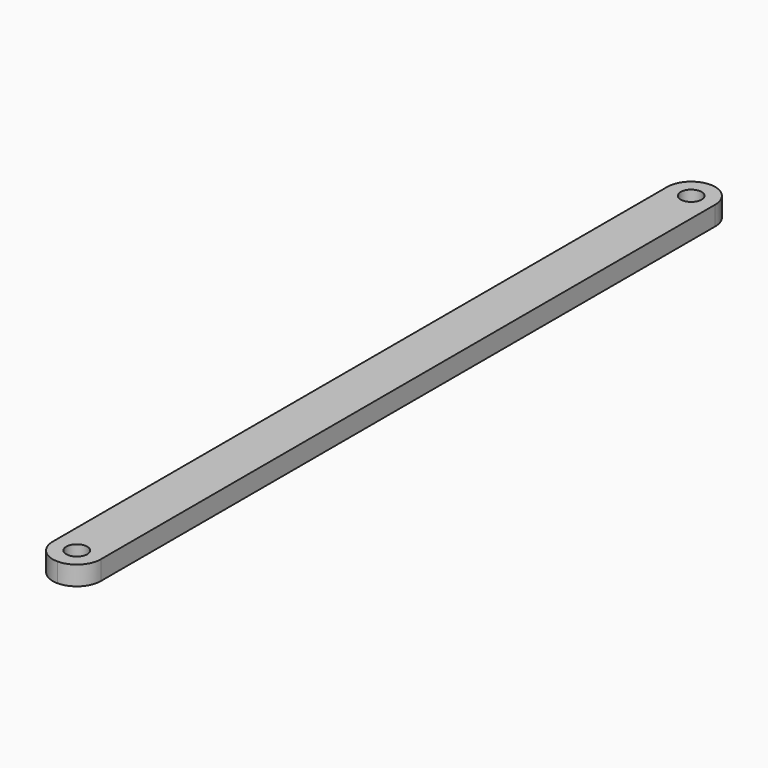
from build123d import *

# Parameters (mm, degrees)
F0_W     = 7.9375
F0_H     = 134.9375
F0_R     = 1.7272
F1_DEPTH = 3.175
F2_R     = 3.96874


# Not quite as in the source:
# - a fillet or chamfer is up to 0.001 mm smaller than in the source, because OpenCascade refuses the exact size


with BuildPart() as f1:
    # F0 (on Top) → F1 (new body)
    with BuildSketch(Plane.XY):
        with Locations((3.96875, -67.46875)):
            Rectangle(F0_W, F0_H)
        with Locations((3.96875, -130.96875)):
            Circle(F0_R, mode=Mode.SUBTRACT)
        with Locations((3.96875, -3.96875)):
            Circle(F0_R, mode=Mode.SUBTRACT)
    extrude(amount=F1_DEPTH)

    # F2 (radius 3.96875 in the source; OpenCascade refuses exactly that, so slightly less here)
    f2_edges = [f1.edges().sort_by_distance(p)[0] for p in [
        (7.9375, 0, 1.5875),
        (0, 0, 1.5875),
        (0, -134.9375, 1.5875),
        (7.9375, -134.9375, 1.5875),
    ]]
    fillet(f2_edges, radius=F2_R)


solid = f1.part
